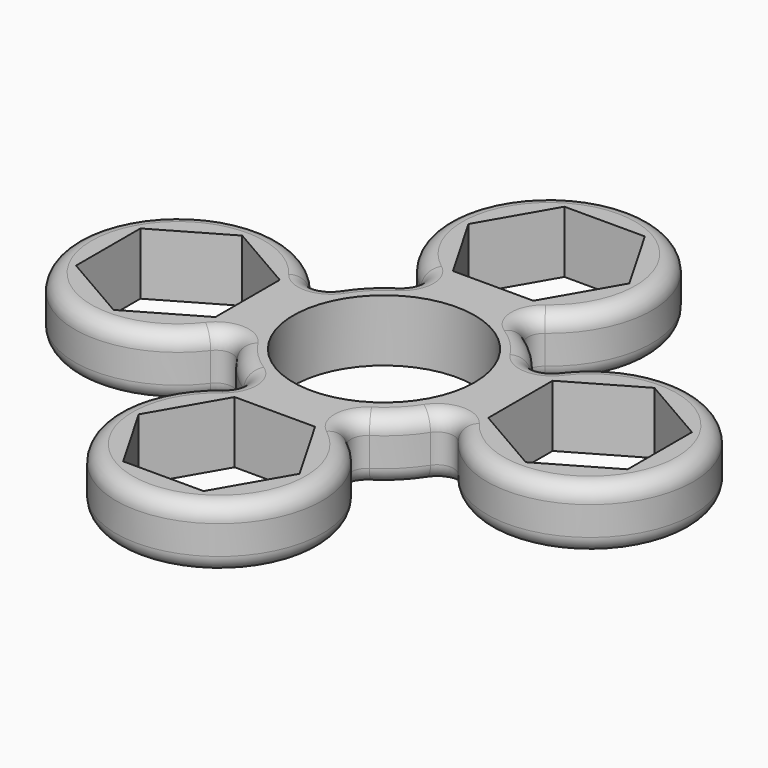
from build123d import *

# Parameters (mm, degrees)
F0_R     = 11
F1_DEPTH = 7.5
F2_R     = 2


# Not quite as in the source:
# - two fillets or chamfers of one size are made in one step


with BuildPart() as f1:
    # F0 (on Top) → F1 (new body)
    with BuildSketch(Plane.XY):
        with BuildLine():
            ThreePointArc((-13.295, 4.3866815476), (-37.5, 0), (-13.295, -4.3866815476))
            ThreePointArc((-13.295, -4.3866815476), (-9.8994949366, -9.8994949366), (-4.3866815476, -13.295))
            ThreePointArc((-4.3866815476, -13.295), (0, -37.5), (4.3866815476, -13.295))
            ThreePointArc((4.3866815476, -13.295), (9.8994949366, -9.8994949366), (13.295, -4.3866815476))
            ThreePointArc((13.295, -4.3866815476), (37.5, 0), (13.295, 4.3866815476))
            ThreePointArc((13.295, 4.3866815476), (9.8994949366, 9.8994949366), (4.3866815476, 13.295))
            ThreePointArc((4.3866815476, 13.295), (0, 37.5), (-4.3866815476, 13.295))
            ThreePointArc((-4.3866815476, 13.295), (-9.8994949366, 9.8994949366), (-13.295, 4.3866815476))
        make_face()
        Polygon((-9.7572195493, -25), (-4.8786097747, -16.55), (4.8786097747, -16.55), (9.7572195493, -25), (4.8786097747, -33.45), (-4.8786097747, -33.45), align=None, mode=Mode.SUBTRACT)
        Polygon((-25, 9.7572195493), (-16.55, 4.8786097747), (-16.55, -4.8786097747), (-25, -9.7572195493), (-33.45, -4.8786097747), (-33.45, 4.8786097747), align=None, mode=Mode.SUBTRACT)
        Circle(F0_R, mode=Mode.SUBTRACT)
        Polygon((16.55, 4.8786097747), (25, 9.7572195493), (33.45, 4.8786097747), (33.45, -4.8786097747), (25, -9.7572195493), (16.55, -4.8786097747), align=None, mode=Mode.SUBTRACT)
        Polygon((-9.7572195493, 25), (-4.8786097747, 33.45), (4.8786097747, 33.45), (9.7572195493, 25), (4.8786097747, 16.55), (-4.8786097747, 16.55), align=None, mode=Mode.SUBTRACT)
    extrude(amount=F1_DEPTH)

    # F2
    f2_edges = [f1.edges().sort_by_distance(p)[0] for p in [
        (-13.295, -4.386682, 3.75),
        (13.295, 4.386682, 3.75),
        (4.386682, -13.295, 3.75),
        (-4.386682, 13.295, 3.75),
        (-13.295, 4.386682, 3.75),
        (-9.899495, 9.899495, 0),
        (-9.899495, 9.899495, 7.5),
        (-37.5, 0, 0),
        (-37.5, 0, 7.5),
        (-4.386682, -13.295, 3.75),
        (-9.899495, -9.899495, 0),
        (-9.899495, -9.899495, 7.5),
        (0, -37.5, 0),
        (0, -37.5, 7.5),
        (13.295, -4.386682, 3.75),
        (9.899495, -9.899495, 0),
        (9.899495, -9.899495, 7.5),
        (37.5, 0, 0),
        (37.5, 0, 7.5),
        (4.386682, 13.295, 3.75),
        (9.899495, 9.899495, 0),
        (9.899495, 9.899495, 7.5),
        (0, 37.5, 0),
        (0, 37.5, 7.5),
    ]]
    fillet(f2_edges, radius=F2_R)


solid = f1.part
